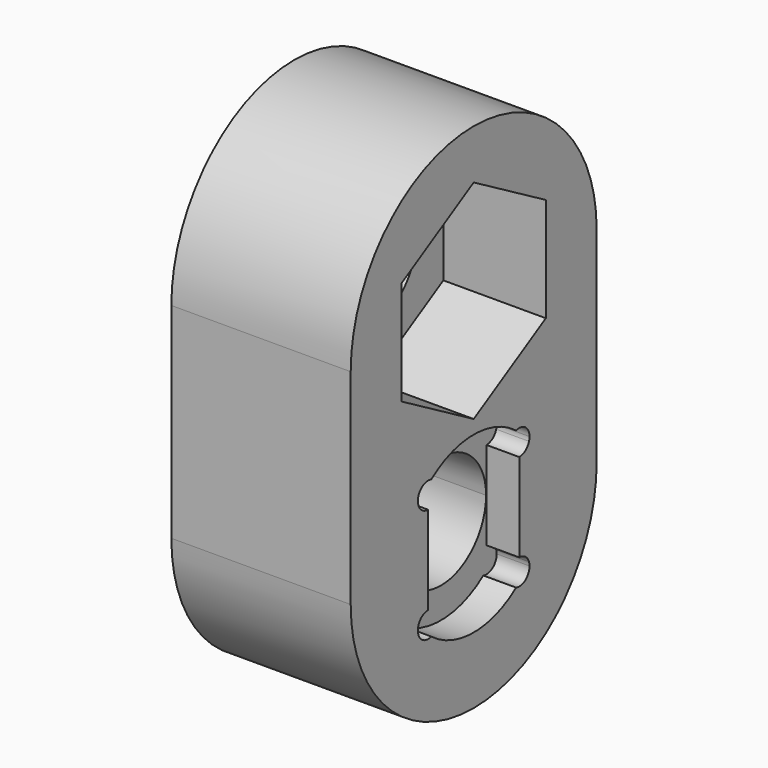
from build123d import *

# Parameters (mm, degrees)
F1_DEPTH = 5.55752
F2_R     = 1.75
F3_DEPTH = 1.016
F4_R     = 1.75
F5_DEPTH = 1.016
F6_DEPTH = 3.175
F7_SIZE  = 1.5875


# Not quite as in the source:
# - a feature names something its author has since deleted; it is built from what else it names


with BuildPart() as f1:
    # F0 (on Right) → F1 (new body)
    with BuildSketch(Plane.YZ):
        with BuildLine():
            ThreePointArc((0.636344373, -4.7197957677), (2.2310225415, -4.2076055743), (3.5497579143, -3.175))
            ThreePointArc((3.5497579143, -3.175), (2.2310225415, -2.1423944257), (0.636344373, -1.6302042323))
            ThreePointArc((0.636344373, -1.6302042323), (0, -1.75), (-0.636344373, -1.6302042323))
            ThreePointArc((-0.636344373, -1.6302042323), (-2.2310225415, -2.1423944257), (-3.5497579143, -3.175))
            ThreePointArc((-3.5497579143, -3.175), (-2.2310225415, -4.2076055743), (-0.636344373, -4.7197957677))
            ThreePointArc((-0.636344373, -4.7197957677), (0, -4.6), (0.636344373, -4.7197957677))
        make_face()
        with BuildLine():
            ThreePointArc((3.5497579143, -3.175), (4.4489958596, -1.6993652025), (4.7625, 0))
            ThreePointArc((4.7625, 0), (0, 4.7625), (-4.7625, 0))
            ThreePointArc((-4.7625, 0), (-4.4489958596, -1.6993652025), (-3.5497579143, -3.175))
            ThreePointArc((-3.5497579143, -3.175), (-2.2310225415, -2.1423944257), (-0.636344373, -1.6302042323))
            ThreePointArc((-0.636344373, -1.6302042323), (-0.9871416685, 1.4450091094), (1.75, 0))
            ThreePointArc((1.75, 0), (1.4450091094, -0.9871416685), (0.636344373, -1.6302042323))
            ThreePointArc((0.636344373, -1.6302042323), (2.2310225415, -2.1423944257), (3.5497579143, -3.175))
        make_face()
        with BuildLine():
            Line((4.7625, -6.35), (4.7625, 0))
            ThreePointArc((4.7625, 0), (4.4489958596, -1.6993652025), (3.5497579143, -3.175))
            ThreePointArc((3.5497579143, -3.175), (4.4489958596, -4.6506347975), (4.7625, -6.35))
        make_face()
        with BuildLine():
            ThreePointArc((4.7625, -6.35), (4.4489958596, -4.6506347975), (3.5497579143, -3.175))
            ThreePointArc((3.5497579143, -3.175), (2.2310225415, -4.2076055743), (0.636344373, -4.7197957677))
            ThreePointArc((0.636344373, -4.7197957677), (1.4450091094, -5.3628583315), (1.75, -6.35))
            ThreePointArc((1.75, -6.35), (-0.9871416685, -7.7950091094), (-0.636344373, -4.7197957677))
            ThreePointArc((-0.636344373, -4.7197957677), (-2.2310225415, -4.2076055743), (-3.5497579143, -3.175))
            ThreePointArc((-3.5497579143, -3.175), (-4.4489958596, -4.6506347975), (-4.7625, -6.35))
            ThreePointArc((-4.7625, -6.35), (0, -11.1125), (4.7625, -6.35))
        make_face()
        with BuildLine():
            ThreePointArc((-3.5497579143, -3.175), (-4.4489958596, -1.6993652025), (-4.7625, 0))
            Line((-4.7625, 0), (-4.7625, -6.35))
            ThreePointArc((-4.7625, -6.35), (-4.4489958596, -4.6506347975), (-3.5497579143, -3.175))
        make_face()
    extrude(amount=F1_DEPTH)

    # F2 (on face) → F3 (cut)
    with BuildSketch(Plane.YZ.offset(5.55752)):
        with BuildLine():
            ThreePointArc((1.368425, -4.5847), (1.4846669962, -4.8653330038), (1.7653, -4.981575))
            Line((1.7653, -4.981575), (1.7653, -4.5847))
            Line((1.7653, -4.5847), (1.368425, -4.5847))
        make_face()
        with BuildLine():
            Line((1.7653, -4.5847), (1.7653, -4.981575))
            ThreePointArc((1.7653, -4.981575), (1.9986038099, -4.9057593371), (2.1427708235, -4.7072787218))
            ThreePointArc((2.1427708235, -4.7072787218), (1.9091883092, -4.4408116908), (1.6427212782, -4.2072291765))
            ThreePointArc((1.6427212782, -4.2072291765), (1.4442406629, -4.3513961901), (1.368425, -4.5847))
            Line((1.368425, -4.5847), (1.7653, -4.5847))
        make_face()
        with BuildLine():
            ThreePointArc((1.7653, -7.718425), (1.4846669962, -7.8346669962), (1.368425, -8.1153))
            Line((1.368425, -8.1153), (1.7653, -8.1153))
            Line((1.7653, -8.1153), (1.7653, -7.718425))
        make_face()
        with BuildLine():
            Line((1.7653, -8.1153), (1.368425, -8.1153))
            ThreePointArc((1.368425, -8.1153), (1.4442406629, -8.3486038099), (1.6427212782, -8.4927708235))
            ThreePointArc((1.6427212782, -8.4927708235), (1.9091883092, -8.2591883092), (2.1427708235, -7.9927212782))
            ThreePointArc((2.1427708235, -7.9927212782), (1.9986038099, -7.7942406629), (1.7653, -7.718425))
            Line((1.7653, -7.718425), (1.7653, -8.1153))
        make_face()
        with BuildLine():
            Line((-1.368425, -8.1153), (-1.7653, -8.1153))
            Line((-1.7653, -8.1153), (-1.7653, -7.718425))
            ThreePointArc((-1.7653, -7.718425), (-1.9986038099, -7.7942406629), (-2.1427708235, -7.9927212782))
            ThreePointArc((-2.1427708235, -7.9927212782), (-1.9091883092, -8.2591883092), (-1.6427212782, -8.4927708235))
            ThreePointArc((-1.6427212782, -8.4927708235), (-1.4442406629, -8.3486038099), (-1.368425, -8.1153))
        make_face()
        with BuildLine():
            Line((-1.7653, -7.718425), (-1.7653, -8.1153))
            Line((-1.7653, -8.1153), (-1.368425, -8.1153))
            ThreePointArc((-1.368425, -8.1153), (-1.4846669962, -7.8346669962), (-1.7653, -7.718425))
        make_face()
        with BuildLine():
            Line((-1.7653, -4.5847), (-1.7653, -4.981575))
            ThreePointArc((-1.7653, -4.981575), (-1.4846669962, -4.8653330038), (-1.368425, -4.5847))
            Line((-1.368425, -4.5847), (-1.7653, -4.5847))
        make_face()
        with BuildLine():
            ThreePointArc((-2.1427708235, -4.7072787218), (-1.9986038099, -4.9057593371), (-1.7653, -4.981575))
            Line((-1.7653, -4.981575), (-1.7653, -4.5847))
            Line((-1.7653, -4.5847), (-1.368425, -4.5847))
            ThreePointArc((-1.368425, -4.5847), (-1.4442406629, -4.3513961901), (-1.6427212782, -4.2072291765))
            ThreePointArc((-1.6427212782, -4.2072291765), (-1.9091883092, -4.4408116908), (-2.1427708235, -4.7072787218))
        make_face()
        with BuildLine():
            ThreePointArc((-1.7653, -7.718425), (-1.4846669962, -7.8346669962), (-1.368425, -8.1153))
            Line((-1.368425, -8.1153), (1.368425, -8.1153))
            ThreePointArc((1.368425, -8.1153), (1.4846669962, -7.8346669962), (1.7653, -7.718425))
            Line((1.7653, -7.718425), (1.7653, -4.981575))
            ThreePointArc((1.7653, -4.981575), (1.4846669962, -4.8653330038), (1.368425, -4.5847))
            Line((1.368425, -4.5847), (-1.368425, -4.5847))
            ThreePointArc((-1.368425, -4.5847), (-1.4846669962, -4.8653330038), (-1.7653, -4.981575))
            Line((-1.7653, -4.981575), (-1.7653, -7.718425))
        make_face()
        with Locations((0, -6.35)):
            Circle(F2_R, mode=Mode.SUBTRACT)
        with BuildLine():
            ThreePointArc((-1.6427212782, -4.2072291765), (-2.0459330038, -4.3040669962), (-2.1427708235, -4.7072787218))
            ThreePointArc((-2.1427708235, -4.7072787218), (-1.9091883092, -4.4408116908), (-1.6427212782, -4.2072291765))
        make_face()
        with BuildLine():
            ThreePointArc((1.6427212782, -4.2072291765), (1.9091883092, -4.4408116908), (2.1427708235, -4.7072787218))
            ThreePointArc((2.1427708235, -4.7072787218), (2.1572939405, -4.6467525283), (2.162175, -4.5847))
            ThreePointArc((2.162175, -4.5847), (1.9986038099, -4.2636406629), (1.6427212782, -4.2072291765))
        make_face()
        with BuildLine():
            ThreePointArc((2.1427708235, -7.9927212782), (1.9091883092, -8.2591883092), (1.6427212782, -8.4927708235))
            ThreePointArc((1.6427212782, -8.4927708235), (1.9986038099, -8.4363593371), (2.162175, -8.1153))
            ThreePointArc((2.162175, -8.1153), (2.1572939405, -8.0532474717), (2.1427708235, -7.9927212782))
        make_face()
        with BuildLine():
            ThreePointArc((-2.1427708235, -7.9927212782), (-2.0459330038, -8.3959330038), (-1.6427212782, -8.4927708235))
            ThreePointArc((-1.6427212782, -8.4927708235), (-1.9091883092, -8.2591883092), (-2.1427708235, -7.9927212782))
        make_face()
        with BuildLine():
            ThreePointArc((-1.6427212782, -4.2072291765), (-1.4442406629, -4.3513961901), (-1.368425, -4.5847))
            Line((-1.368425, -4.5847), (1.368425, -4.5847))
            ThreePointArc((1.368425, -4.5847), (1.4442406629, -4.3513961901), (1.6427212782, -4.2072291765))
            ThreePointArc((1.6427212782, -4.2072291765), (0, -3.65), (-1.6427212782, -4.2072291765))
        make_face()
        with BuildLine():
            Line((1.368425, -8.1153), (-1.368425, -8.1153))
            ThreePointArc((-1.368425, -8.1153), (-1.4442406629, -8.3486038099), (-1.6427212782, -8.4927708235))
            ThreePointArc((-1.6427212782, -8.4927708235), (0, -9.05), (1.6427212782, -8.4927708235))
            ThreePointArc((1.6427212782, -8.4927708235), (1.4442406629, -8.3486038099), (1.368425, -8.1153))
        make_face()
    extrude(amount=-F3_DEPTH, mode=Mode.SUBTRACT)

    # F4 (on face) → F5 (cut)
    with BuildSketch(Plane(origin=(0, 0, 0), x_dir=(0, -1, 0), z_dir=(-1, 0, 0))):
        with BuildLine():
            ThreePointArc((1.7653, -1.368425), (1.4846669962, -1.4846669962), (1.368425, -1.7653))
            Line((1.368425, -1.7653), (1.7653, -1.7653))
            Line((1.7653, -1.7653), (1.7653, -1.368425))
        make_face()
        with BuildLine():
            Line((1.7653, -1.7653), (1.368425, -1.7653))
            ThreePointArc((1.368425, -1.7653), (1.4442406629, -1.9986038099), (1.6427212782, -2.1427708235))
            ThreePointArc((1.6427212782, -2.1427708235), (1.9091883092, -1.9091883092), (2.1427708235, -1.6427212782))
            ThreePointArc((2.1427708235, -1.6427212782), (1.9986038099, -1.4442406629), (1.7653, -1.368425))
            Line((1.7653, -1.368425), (1.7653, -1.7653))
        make_face()
        with BuildLine():
            Line((-1.7653, -1.368425), (-1.7653, -1.7653))
            Line((-1.7653, -1.7653), (-1.368425, -1.7653))
            ThreePointArc((-1.368425, -1.7653), (-1.4846669962, -1.4846669962), (-1.7653, -1.368425))
        make_face()
        with BuildLine():
            Line((-1.368425, -1.7653), (-1.7653, -1.7653))
            Line((-1.7653, -1.7653), (-1.7653, -1.368425))
            ThreePointArc((-1.7653, -1.368425), (-1.9986038099, -1.4442406629), (-2.1427708235, -1.6427212782))
            ThreePointArc((-2.1427708235, -1.6427212782), (-1.9091883092, -1.9091883092), (-1.6427212782, -2.1427708235))
            ThreePointArc((-1.6427212782, -2.1427708235), (-1.4442406629, -1.9986038099), (-1.368425, -1.7653))
        make_face()
        with BuildLine():
            Line((-1.7653, 1.7653), (-1.7653, 1.368425))
            ThreePointArc((-1.7653, 1.368425), (-1.4846669962, 1.4846669962), (-1.368425, 1.7653))
            Line((-1.368425, 1.7653), (-1.7653, 1.7653))
        make_face()
        with BuildLine():
            ThreePointArc((-2.1427708235, 1.6427212782), (-1.9986038099, 1.4442406629), (-1.7653, 1.368425))
            Line((-1.7653, 1.368425), (-1.7653, 1.7653))
            Line((-1.7653, 1.7653), (-1.368425, 1.7653))
            ThreePointArc((-1.368425, 1.7653), (-1.4442406629, 1.9986038099), (-1.6427212782, 2.1427708235))
            ThreePointArc((-1.6427212782, 2.1427708235), (-1.9091883092, 1.9091883092), (-2.1427708235, 1.6427212782))
        make_face()
        with BuildLine():
            ThreePointArc((1.368425, 1.7653), (1.4846669962, 1.4846669962), (1.7653, 1.368425))
            Line((1.7653, 1.368425), (1.7653, 1.7653))
            Line((1.7653, 1.7653), (1.368425, 1.7653))
        make_face()
        with BuildLine():
            Line((1.7653, 1.7653), (1.7653, 1.368425))
            ThreePointArc((1.7653, 1.368425), (1.9986038099, 1.4442406629), (2.1427708235, 1.6427212782))
            ThreePointArc((2.1427708235, 1.6427212782), (1.9091883092, 1.9091883092), (1.6427212782, 2.1427708235))
            ThreePointArc((1.6427212782, 2.1427708235), (1.4442406629, 1.9986038099), (1.368425, 1.7653))
            Line((1.368425, 1.7653), (1.7653, 1.7653))
        make_face()
        with BuildLine():
            ThreePointArc((-1.7653, -1.368425), (-1.4846669962, -1.4846669962), (-1.368425, -1.7653))
            Line((-1.368425, -1.7653), (1.368425, -1.7653))
            ThreePointArc((1.368425, -1.7653), (1.4846669962, -1.4846669962), (1.7653, -1.368425))
            Line((1.7653, -1.368425), (1.7653, 1.368425))
            ThreePointArc((1.7653, 1.368425), (1.4846669962, 1.4846669962), (1.368425, 1.7653))
            Line((1.368425, 1.7653), (-1.368425, 1.7653))
            ThreePointArc((-1.368425, 1.7653), (-1.4846669962, 1.4846669962), (-1.7653, 1.368425))
            Line((-1.7653, 1.368425), (-1.7653, -1.368425))
        make_face()
        Circle(F4_R, mode=Mode.SUBTRACT)
        with BuildLine():
            ThreePointArc((-1.6427212782, 2.1427708235), (-2.0459330038, 2.0459330038), (-2.1427708235, 1.6427212782))
            ThreePointArc((-2.1427708235, 1.6427212782), (-1.9091883092, 1.9091883092), (-1.6427212782, 2.1427708235))
        make_face()
        with BuildLine():
            ThreePointArc((-2.1427708235, -1.6427212782), (-2.0459330038, -2.0459330038), (-1.6427212782, -2.1427708235))
            ThreePointArc((-1.6427212782, -2.1427708235), (-1.9091883092, -1.9091883092), (-2.1427708235, -1.6427212782))
        make_face()
        with BuildLine():
            ThreePointArc((2.1427708235, -1.6427212782), (1.9091883092, -1.9091883092), (1.6427212782, -2.1427708235))
            ThreePointArc((1.6427212782, -2.1427708235), (1.9986038099, -2.0863593371), (2.162175, -1.7653))
            ThreePointArc((2.162175, -1.7653), (2.1572939405, -1.7032474717), (2.1427708235, -1.6427212782))
        make_face()
        with BuildLine():
            ThreePointArc((1.6427212782, 2.1427708235), (1.9091883092, 1.9091883092), (2.1427708235, 1.6427212782))
            ThreePointArc((2.1427708235, 1.6427212782), (2.1572939405, 1.7032474717), (2.162175, 1.7653))
            ThreePointArc((2.162175, 1.7653), (1.9986038099, 2.0863593371), (1.6427212782, 2.1427708235))
        make_face()
        with BuildLine():
            ThreePointArc((-1.6427212782, 2.1427708235), (-1.4442406629, 1.9986038099), (-1.368425, 1.7653))
            Line((-1.368425, 1.7653), (1.368425, 1.7653))
            ThreePointArc((1.368425, 1.7653), (1.4442406629, 1.9986038099), (1.6427212782, 2.1427708235))
            ThreePointArc((1.6427212782, 2.1427708235), (0, 2.7), (-1.6427212782, 2.1427708235))
        make_face()
        with BuildLine():
            Line((1.368425, -1.7653), (-1.368425, -1.7653))
            ThreePointArc((-1.368425, -1.7653), (-1.4442406629, -1.9986038099), (-1.6427212782, -2.1427708235))
            ThreePointArc((-1.6427212782, -2.1427708235), (0, -2.7), (1.6427212782, -2.1427708235))
            ThreePointArc((1.6427212782, -2.1427708235), (1.4442406629, -1.9986038099), (1.368425, -1.7653))
        make_face()
    extrude(amount=-F5_DEPTH, mode=Mode.SUBTRACT)

    # F2 (on face) → F6 (cut)
    with BuildSketch(Plane.YZ.offset(5.55752)):
        Polygon((-2.794, -1.6131166521), (0, -3.2262333042), (2.794, -1.6131166521), (2.794, 1.6131166521), (0, 3.2262333042), (-2.794, 1.6131166521), align=None)
        Circle(F2_R, mode=Mode.SUBTRACT)
    extrude(amount=-F6_DEPTH, mode=Mode.SUBTRACT)

    # F7
    f7_edges = [f1.edges().sort_by_distance(p)[0] for p in [
        (0, -0.636344, -7.980204),
    ]]
    chamfer(f7_edges, length=F7_SIZE)


solid = f1.part
